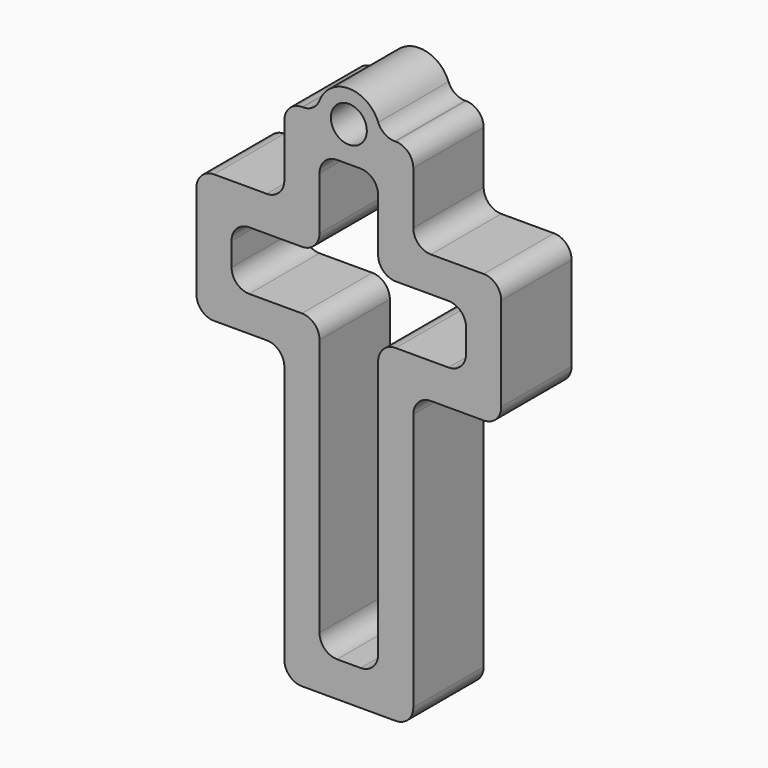
from build123d import *

# Parameters (mm, degrees)
F1_DEPTH = 15
F2_R     = 3
F3_R     = 3
F4_R     = 3


with BuildPart() as f1:
    # F0 (on Front) → F1 (new body)
    with BuildSketch(Plane.XZ):
        with BuildLine():
            Line((-16, 27.1340573728), (-16, -16.8659426272))
            Line((-16, -16.8659426272), (-16, -22.8659426272))
            Line((-16, -22.8659426272), (6, -22.8659426272))
            Line((6, -22.8659426272), (6, 27.1340573728))
            Line((6, 27.1340573728), (15, 27.1340573728))
            Line((15, 27.1340573728), (21, 27.1340573728))
            Line((21, 27.1340573728), (21, 49.1340573728))
            Line((21, 49.1340573728), (6, 49.1340573728))
            Line((6, 49.1340573728), (6, 64.1340573728))
            Line((6, 64.1340573728), (0.3713240896, 64.1340573728))
            ThreePointArc((0.3713240896, 64.1340573728), (-5, 58.7627332832), (-10.3713240896, 64.1340573728))
            Line((-10.3713240896, 64.1340573728), (-16, 64.1340573728))
            Line((-16, 64.1340573728), (-16, 49.1340573728))
            Line((-16, 49.1340573728), (-31, 49.1340573728))
            Line((-31, 49.1340573728), (-31, 27.1340573728))
            Line((-31, 27.1340573728), (-25, 27.1340573728))
            Line((-25, 27.1340573728), (-16, 27.1340573728))
        make_face()
        Polygon((-10, 58.1340573728), (0, 58.1340573728), (0, 43.1340573728), (15, 43.1340573728), (15, 33.1340573728), (0, 33.1340573728), (0, -16.8659426272), (-10, -16.8659426272), (-10, 33.1340573728), (-25, 33.1340573728), (-25, 43.1340573728), (-10, 43.1340573728), align=None, mode=Mode.SUBTRACT)
        with BuildLine():
            ThreePointArc((0.3713240896, 64.1340573728), (-5, 69.5053814624), (-10.3713240896, 64.1340573728))
            Line((-10.3713240896, 64.1340573728), (-8.0673756686, 64.1340573728))
            ThreePointArc((-8.0673756686, 64.1340573728), (-5, 67.2014330414), (-1.9326243314, 64.1340573728))
            Line((-1.9326243314, 64.1340573728), (0.3713240896, 64.1340573728))
        make_face()
        with BuildLine():
            Line((-8.0673756686, 64.1340573728), (-10.3713240896, 64.1340573728))
            ThreePointArc((-10.3713240896, 64.1340573728), (-5, 58.7627332832), (0.3713240896, 64.1340573728))
            Line((0.3713240896, 64.1340573728), (-1.9326243314, 64.1340573728))
            ThreePointArc((-1.9326243314, 64.1340573728), (-5, 61.0666817042), (-8.0673756686, 64.1340573728))
        make_face()
    extrude(amount=F1_DEPTH)

    # F2
    f2_edges = [f1.edges().sort_by_distance(p)[0] for p in [
        (-10, -7.5, -16.865943),
        (-10, -7.5, 33.134057),
        (-25, -7.5, 33.134057),
        (0, -7.5, -16.865943),
        (0, -7.5, 33.134057),
        (15, -7.5, 33.134057),
        (15, -7.5, 43.134057),
        (0, -7.5, 43.134057),
        (0, -7.5, 58.134057),
        (-10, -7.5, 58.134057),
        (-10, -7.5, 43.134057),
        (-25, -7.5, 43.134057),
    ]]
    fillet(f2_edges, radius=F2_R)

    # F3
    f3_edges = [f1.edges().sort_by_distance(p)[0] for p in [
        (6, -7.5, 49.134057),
    ]]
    fillet(f3_edges, radius=F3_R)

    # F4
    f4_edges = [f1.edges().sort_by_distance(p)[0] for p in [
        (6, -7.5, 64.134057),
        (0.371324, -7.5, 64.134057),
        (21, -7.5, 27.134057),
        (6, -7.5, 27.134057),
        (6, -7.5, -22.865943),
        (-16, -7.5, -22.865943),
        (-16, -7.5, 27.134057),
        (-31, -7.5, 27.134057),
        (-10.371324, -7.5, 64.134057),
        (-16, -7.5, 64.134057),
        (-16, -7.5, 49.134057),
        (21, -7.5, 49.134057),
        (-31, -7.5, 49.134057),
    ]]
    fillet(f4_edges, radius=F4_R)


solid = f1.part
